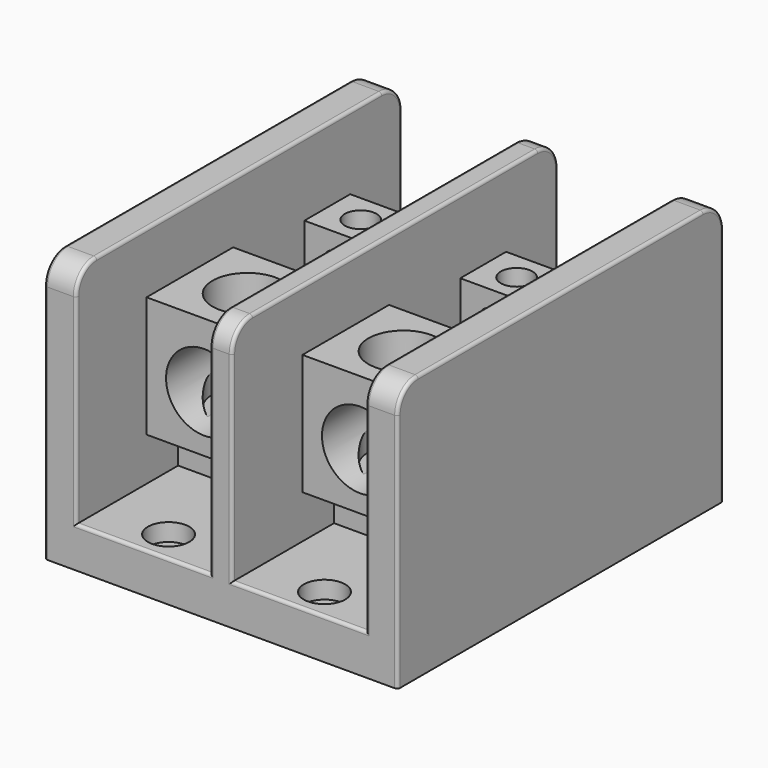
from build123d import *

# Parameters (mm, degrees)
F0_W      = 88.10625
F0_H      = 101.6
F1_DEPTH  = 10.16
F2_R      = 2.54
F3_DEPTH  = 10.16
F4_R      = 5.159375
F5_DEPTH  = 4.365625
F6_W      = 33.3375
F6_H      = 38.1
F7_DEPTH  = 12.7
F8_W      = 7.9375
F8_H      = 101.6
F8_W_2    = 5.55625
F9_DEPTH  = 56.118125
F10_W     = 28.7734375
F10_H     = 63.5
F11_DEPTH = 30.1625
F12_W     = 28.7734375
F12_H     = 22.225
F13_DEPTH = 15.478125
F14_DEPTH = 3.175
F15_R     = 8.73125
F16_DEPTH = 25.003125
F17_R     = 9.525
F18_DEPTH = 27.94
F19_R     = 2.667
F19_R_2   = 3.96875
F20_DEPTH = 11.90625
F21_DEPTH = 14.684375
F22_R     = 3.96875
F23_DEPTH = 11.509375
F24_R     = 3.96875
F25_DEPTH = 14.732
F26_DEPTH = 10.668
F28_R     = 6.35
F29_R     = 0.762


with BuildPart() as f1:
    # F0 (on Top) → F1 (new body)
    with BuildSketch(Plane.XY):
        Rectangle(F0_W, F0_H)
    extrude(amount=F1_DEPTH)

    # F2 (on face) → F3 (cut)
    with BuildSketch(Plane.XY.offset(10.16)):
        with Locations((-19.446875, 42.8625)):
            Circle(F2_R)
        with Locations((19.446875, 42.8625)):
            Circle(F2_R)
        with Locations((-19.446875, -42.8625)):
            Circle(F2_R)
        with Locations((19.446875, -42.8625)):
            Circle(F2_R)
    extrude(amount=-F3_DEPTH, mode=Mode.SUBTRACT)

    # F4 (on face) → F5 (cut)
    with BuildSketch(Plane.XY.offset(10.16)):
        with Locations((-19.446875, 42.8625)):
            Circle(F4_R)
        with Locations((19.446875, 42.8625)):
            Circle(F4_R)
        with Locations((-19.446875, -42.8625)):
            Circle(F4_R)
        with Locations((19.446875, -42.8625)):
            Circle(F4_R)
    extrude(amount=-F5_DEPTH, mode=Mode.SUBTRACT)

    # F6 (on face) → F7 (join)
    with BuildSketch(Plane.XY.offset(10.16)):
        with Locations((-19.446875, 0)):
            Rectangle(F6_W, F6_H)
        with Locations((19.446875, 0)):
            Rectangle(F6_W, F6_H)
    extrude(amount=F7_DEPTH)

    # F8 (on face) → F9 (join)
    with BuildSketch(Plane.XY.offset(10.16)):
        with Locations((-40.084375, 0)):
            Rectangle(F8_W, F8_H)
        Rectangle(F8_W_2, F8_H)
        with Locations((40.084375, 0)):
            Rectangle(F8_W, F8_H)
    extrude(amount=F9_DEPTH)

    # F28
    f28_edges = [f1.edges().sort_by_distance(p)[0] for p in [
        (-40.084375, 50.8, 66.278125),
        (0, 50.8, 66.278125),
        (40.084375, 50.8, 66.278125),
        (-40.084375, -50.8, 66.278125),
        (0, -50.8, 66.278125),
        (40.084375, -50.8, 66.278125),
    ]]
    fillet(f28_edges, radius=F28_R)

    # F29
    f29_edges = [f1.edges().sort_by_distance(p)[0] for p in [
        (44.053125, -50.8, 29.964063),
        (36.115625, -50.8, 35.044063),
        (19.446875, -50.8, 10.16),
        (2.778125, -50.8, 35.044063),
        (-2.778125, -50.8, 35.044063),
        (-19.446875, -50.8, 10.16),
        (-36.115625, -50.8, 35.044063),
        (-44.053125, -50.8, 29.964063),
        (-19.446875, 50.8, 10.16),
        (19.446875, 50.8, 10.16),
        (-44.053125, 50.8, 29.964063),
        (-44.053125, 48.940128, 64.418253),
        (-44.053125, 0, 66.278125),
        (-44.053125, -48.940128, 64.418253),
        (44.053125, 50.8, 29.964063),
        (36.115625, 50.8, 35.044063),
        (2.778125, 50.8, 35.044063),
        (-36.115625, 50.8, 35.044063),
        (-2.778125, 50.8, 35.044063),
        (-36.115625, 48.940128, 64.418253),
        (-36.115625, 0, 66.278125),
        (-36.115625, -48.940128, 64.418253),
        (44.053125, -48.940128, 64.418253),
        (44.053125, 0, 66.278125),
        (44.053125, 48.940128, 64.418253),
        (36.115625, 48.940128, 64.418253),
        (36.115625, -48.940128, 64.418253),
        (36.115625, 0, 66.278125),
        (2.778125, 48.940128, 64.418253),
        (2.778125, 0, 66.278125),
        (2.778125, -48.940128, 64.418253),
        (-2.778125, 48.940128, 64.418253),
        (-2.778125, -48.940128, 64.418253),
        (-2.778125, 0, 66.278125),
    ]]
    fillet(f29_edges, radius=F29_R)


with BuildPart() as f11:
    # F10 (on face) → F11 (new body)
    with BuildSketch(Plane.XY.offset(22.86)):
        with Locations((-19.446875, 0)):
            Rectangle(F10_W, F10_H)
    extrude(amount=F11_DEPTH)

    # F12 (on face) → F13 (cut)
    with BuildSketch(Plane.XY.offset(53.0225)):
        with Locations((-19.446875, 6.35)):
            Rectangle(F12_W, F12_H)
    extrude(amount=-F13_DEPTH, mode=Mode.SUBTRACT)

    # F14 (cut): a face of the model
    f14_faces = [f11.faces().sort_by_distance(p)[0] for p in [
        (-19.446875, 24.60625, 53.0225),
    ]]
    extrude(f14_faces, amount=-F14_DEPTH, mode=Mode.SUBTRACT)

    # F15 (on face) → F16 (cut)
    with BuildSketch(Plane.XY.offset(53.0225)):
        with Locations((-19.446875, -18.25625)):
            Circle(F15_R)
    extrude(amount=-F16_DEPTH, mode=Mode.SUBTRACT)

    # F17 (on face) → F18 (cut)
    with BuildSketch(Plane.XZ.offset(31.75)):
        with Locations((-19.446875, 36.83)):
            Circle(F17_R)
    extrude(amount=-F18_DEPTH, mode=Mode.SUBTRACT)

    # F19 (on face) → F20 (cut)
    with BuildSketch(Plane.XY.offset(37.544375)):
        with Locations((-27.48359375, 0.396875)):
            Circle(F19_R)
        with Locations((-11.41015625, 0.396875)):
            Circle(F19_R)
        with Locations((-25.49921875, 12.7)):
            Circle(F19_R_2)
        with Locations((-13.39453125, 12.7)):
            Circle(F19_R_2)
    extrude(amount=-F20_DEPTH, mode=Mode.SUBTRACT)

    # F21 (cut): faces of the model
    f21_faces = [f11.faces().sort_by_distance(p)[0] for p in [
        (-27.48359375, 0.396875, 25.638125),
        (-11.41015625, 0.396875, 25.638125),
    ]]
    extrude(f21_faces, amount=-F21_DEPTH, mode=Mode.SUBTRACT)

    # F22 (on face) → F23 (cut)
    with BuildSketch(Plane.XY.offset(49.8475)):
        with Locations((-25.49921875, 24.60625)):
            Circle(F22_R)
        with Locations((-13.39453125, 24.60625)):
            Circle(F22_R)
    extrude(amount=-F23_DEPTH, mode=Mode.SUBTRACT)

    # F24 (on face) → F25 (cut)
    with BuildSketch(Plane(origin=(0, 31.75, 0), x_dir=(-1, 0, 0), z_dir=(0, 1, 0))):
        with Locations((13.39453125, 41.91)):
            Circle(F24_R)
        with Locations((25.49921875, 41.91)):
            Circle(F24_R)
        with Locations((13.39453125, 29.21)):
            Circle(F24_R)
        with Locations((25.49921875, 29.21)):
            Circle(F24_R)
    extrude(amount=-F25_DEPTH, mode=Mode.SUBTRACT)

    # F26 (cut): faces of the model
    f26_faces = [f11.faces().sort_by_distance(p)[0] for p in [
        (-13.39453125, 17.018, 29.21),
        (-25.49921875, 17.018, 29.21),
    ]]
    extrude(f26_faces, amount=-F26_DEPTH, mode=Mode.SUBTRACT)


with BuildPart() as f27_1:
    # F27: copy of F11
    add(f11.part.moved(Location((38.89375, 0, 0))))


solid = Compound([f1.part, f11.part, f27_1.part])
